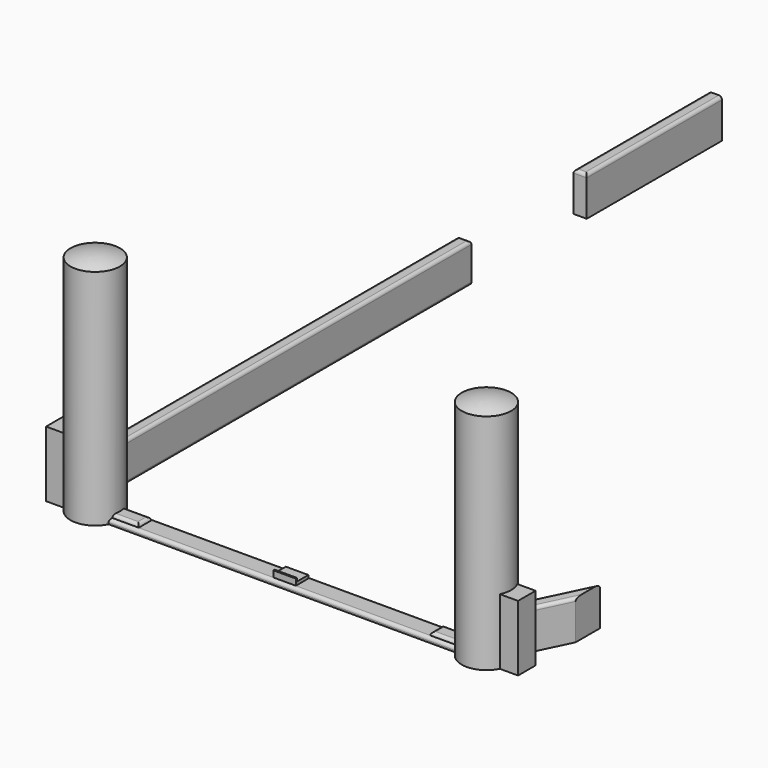
from build123d import *

# Parameters (mm, degrees)
F1_DEPTH  = 12.5
F0_W      = 4.2
F0_H      = 54
F2_DEPTH  = 21
F8_DEPTH  = 1.5
F9_R      = 1
F11_DEPTH = 1
F10_W     = 7.2
F10_H     = 5
F12_R     = 0.99999
F13_R     = 1
F13_2_R   = 1
F14_W     = 7.2
F14_H     = 0.5
F15_DEPTH = 1


# Not quite as in the source:
# - a fillet or chamfer is up to 0.001 mm smaller than in the source, because OpenCascade refuses the exact size


with BuildPart() as f1:
    # F0 (on Top) → F1 (new body)
    with BuildSketch(Plane.XY):
        with BuildLine():
            ThreePointArc((-7.0823724839, 3.5), (-5.3422902804, 5.8197881886), (-2.8823724839, 7.3554013394))
            Line((-2.8823724839, 7.3554013394), (-2.8823724839, 153.9))
            Line((-2.8823724839, 153.9), (-7.0823724839, 153.9))
            Line((-7.0823724839, 153.9), (-7.0823724839, 3.5))
        make_face()
    extrude(amount=F1_DEPTH)

    # F0 (on Top) → F2 (join)
    with BuildSketch(Plane.XY):
        with BuildLine():
            Line((-12.9, -3.5), (-7.0823724839, -3.5))
            ThreePointArc((-7.0823724839, -3.5), (-7.9, 0), (-7.0823724839, 3.5))
            Line((-7.0823724839, 3.5), (-12.9, 3.5))
            Line((-12.9, 3.5), (-12.9, -3.5))
        make_face()
    extrude(amount=F2_DEPTH)

    # F4 (on Right) → F5 (revolve)
    with BuildSketch(Plane.YZ):
        with BuildLine():
            Line((-7.9, 71.3736223973), (-7.9, 0))
            Line((-7.9, 0), (0, 0))
            Line((0, 0), (0, 73))
            ThreePointArc((0, 73), (-4.032837218, 72.5891864041), (-7.9, 71.3736223973))
        make_face()
    revolve(axis=Axis((0, 0, 36.5), (0, 0, 1)))



with BuildPart() as f1b:
    # F0 (on Top) → F1, piece 2 (new body)
    with BuildSketch(Plane.XY):
        with Locations((-4.9823724839, 226.9)):
            Rectangle(F0_W, F0_H)
    extrude(amount=F1_DEPTH)

    # F13#2
    f13_2_edges = [f1b.edges().sort_by_distance(p)[0] for p in [
        (-2.882372, 226.9, 12.5),
        (-7.082372, 226.9, 12.5),
        (-4.982372, 199.9, 12.5),
    ]]
    fillet(f13_2_edges, radius=F13_2_R)


with BuildPart() as f1c:
    # F0 (on Top) → F1, piece 3 (new body)
    with BuildSketch(Plane.XY):
        with BuildLine():
            Line((137.9, 29.1563547549), (127.4451735987, 7.5120653666))
            ThreePointArc((127.4451735987, 7.5120653666), (129.371097675, 6.5805398802), (130.9764612849, 5.1664214413))
            Line((130.9764612849, 5.1664214413), (137.9, 19.5))
            Line((137.9, 19.5), (137.9, 29.1563547549))
        make_face()
    extrude(amount=F1_DEPTH)



with BuildPart() as f2:
    # F0 (on Top) → F2, piece 2 (new body)
    with BuildSketch(Plane.XY):
        with BuildLine():
            ThreePointArc((132.9, 0), (132.6928779602, -1.7971167711), (132.0823724839, -3.5))
            Line((132.0823724839, -3.5), (137.9, -3.5))
            Line((137.9, -3.5), (137.9, 3.5))
            Line((137.9, 3.5), (132.0823724839, 3.5))
            ThreePointArc((132.0823724839, 3.5), (132.6928779602, 1.7971167711), (132.9, 0))
        make_face()
    extrude(amount=F2_DEPTH)


with BuildPart() as f1c_1:
    add(f1c.part)

    add(f2.part)  # F7 merges F2
    # F6 (on plane+point) → F7 (revolve)
    with BuildSketch(Plane.YZ.offset(125)):
        with BuildLine():
            Line((-7.9, 0), (0, 0))
            Line((0, 0), (0, 73))
            ThreePointArc((0, 73), (-4.032837218, 72.5891864041), (-7.9, 71.3736223973))
            Line((-7.9, 71.3736223973), (-7.9, 0))
        make_face()
    revolve(axis=Axis((125, 0, 36.5), (0, 0, 1)))


with BuildPart() as f1_1:
    add(f1.part)

    add(f1c_1.part)  # F8 merges F1c
    # F0 (on Top) → F8 (join)
    with BuildSketch(Plane.XY):
        with BuildLine():
            ThreePointArc((7.0823724839, 3.5), (7.6928779602, 1.7971167711), (7.9, 0))
            ThreePointArc((7.9, 0), (7.6928779602, -1.7971167711), (7.0823724839, -3.5))
            Line((7.0823724839, -3.5), (117.9176275161, -3.5))
            ThreePointArc((117.9176275161, -3.5), (117.1, 0), (117.9176275161, 3.5))
            Line((117.9176275161, 3.5), (7.0823724839, 3.5))
        make_face()
    extrude(amount=F8_DEPTH)

    # F9
    f9_edges = [f1_1.edges().sort_by_distance(p)[0] for p in [
        (62.5, -3.5, 1.5),
        (62.5, 3.5, 1.5),
    ]]
    fillet(f9_edges, radius=F9_R)

    # F10 (on face) → F11 (join)
    with BuildSketch(Plane.XY.offset(1.5)):
        with BuildLine():
            Line((15.9, 2.5), (7.4939975981, 2.5))
            ThreePointArc((7.4939975981, 2.5), (7.9, 0), (7.4939975981, -2.5))
            Line((7.4939975981, -2.5), (15.9, -2.5))
            Line((15.9, -2.5), (15.9, 2.5))
        make_face()
        with BuildLine():
            Line((117.5060024019, 2.5), (109.1, 2.5))
            Line((109.1, 2.5), (109.1, -2.5))
            Line((109.1, -2.5), (117.5060024019, -2.5))
            ThreePointArc((117.5060024019, -2.5), (117.1, 0), (117.5060024019, 2.5))
        make_face()
    extrude(amount=F11_DEPTH)

    # F12 (radius 1 in the source; OpenCascade refuses exactly that, so slightly less here)
    f12_edges = [f1_1.edges().sort_by_distance(p)[0] for p in [
        (11.696999, -2.5, 2.5),
        (15.9, 0, 2.5),
        (11.696999, 2.5, 2.5),
        (113.303001, -2.5, 2.5),
        (109.1, 0, 2.5),
        (113.303001, 2.5, 2.5),
    ]]
    fillet(f12_edges, radius=F12_R)

    # F13
    f13_edges = [f1_1.edges().sort_by_distance(p)[0] for p in [
        (-2.882372, 80.627701, 12.5),
        (-7.082372, 78.7, 12.5),
        (-2.882372, 80.627701, 0),
        (-4.982372, 153.9, 12.5),
        (134.438231, 12.333211, 12.5),
        (132.672587, 18.33421, 12.5),
    ]]
    fillet(f13_edges, radius=F13_R)


with BuildPart() as f11:
    # F10 (on face) → F11, piece 2 (new body)
    with BuildSketch(Plane.XY.offset(1.5)):
        with Locations((62.5, 0)):
            Rectangle(F10_W, F10_H)
    extrude(amount=F11_DEPTH)

    # F14 (on face) → F15 (join)
    with BuildSketch(Plane.XY.offset(2.5)):
        with Locations((62.5, -2.25)):
            Rectangle(F14_W, F14_H)
    extrude(amount=F15_DEPTH)


solid = Compound([f1b.part, f1_1.part, f11.part])
